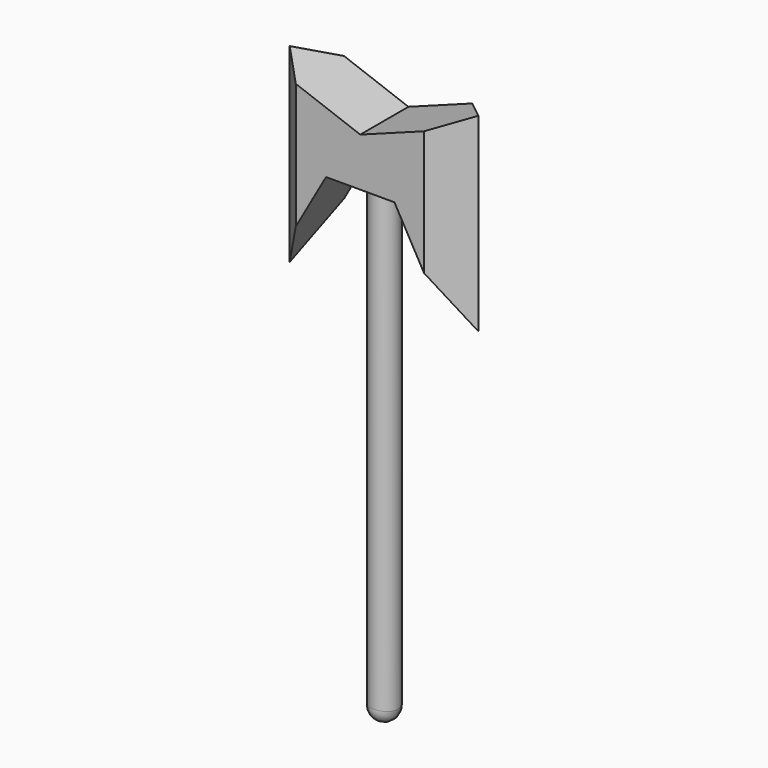
from build123d import *

# Parameters (mm, degrees)
F0_R        = 1.27
F1_DEPTH    = 43.18
F3_DEPTH    = 2.794
F4_T1_DEPTH = 48.6435811926


# Not quite as in the source:
# - a fillet or chamfer that OpenCascade refuses, or shapes differently, is made with other operations: its cross-section is extruded or revolved along the edge and cut away or added


with BuildPart() as f1:
    # F0 (on Top) → F1 (new body)
    with BuildSketch(Plane.XY):
        Circle(F0_R)
    extrude(amount=F1_DEPTH)

    # F5 (on Top) → F6 (revolve)
    with BuildSketch(Plane.XY):
        with BuildLine():
            Line((0, -1.2790904148), (0, 1.2841251446))
            ThreePointArc((0, 1.2841251446), (-1.2710222962, 0.0025173649), (0, -1.2790904148))
        make_face()
    revolve(axis=Axis((0, 0.0025173649, 0), (0, 1, 0)))


with BuildPart() as f3:
    # F2 (on Front) → F3 (new body, symmetric)
    with BuildSketch(Plane.XZ):
        Polygon((-3.1743557192, 43.1767851114), (3.1734784134, 43.1767851114), (10.9989056364, 29.2393378913), (10.9989056364, 51.7546199262), (0, 47.6719401777), (-11.0619841143, 51.7546199262), (-11.0619841143, 29.2393378913), align=None)
    extrude(amount=F3_DEPTH, both=True)

    # F4: chamfer of 5.08 on 4 edges, made by hand

    # F4_s2 → F4_t1 (cut)
    with BuildSketch(Plane.XY.offset(16.1751883125)):
        Polygon((10.9989056364, 2.286), (5.9189056364, -2.794), (10.9989056364, -2.794), align=None)
        Polygon((10.9989056364, -2.286), (5.9189056364, 2.794), (10.9989056364, 2.794), align=None)
        Polygon((-11.0619841143, 2.286), (-5.9819841143, -2.794), (-11.0619841143, -2.794), align=None)
        Polygon((-11.0619841143, -2.286), (-5.9819841143, 2.794), (-11.0619841143, 2.794), align=None)
    extrude(amount=F4_T1_DEPTH, mode=Mode.SUBTRACT)


solid = Compound([f1.part, f3.part])
